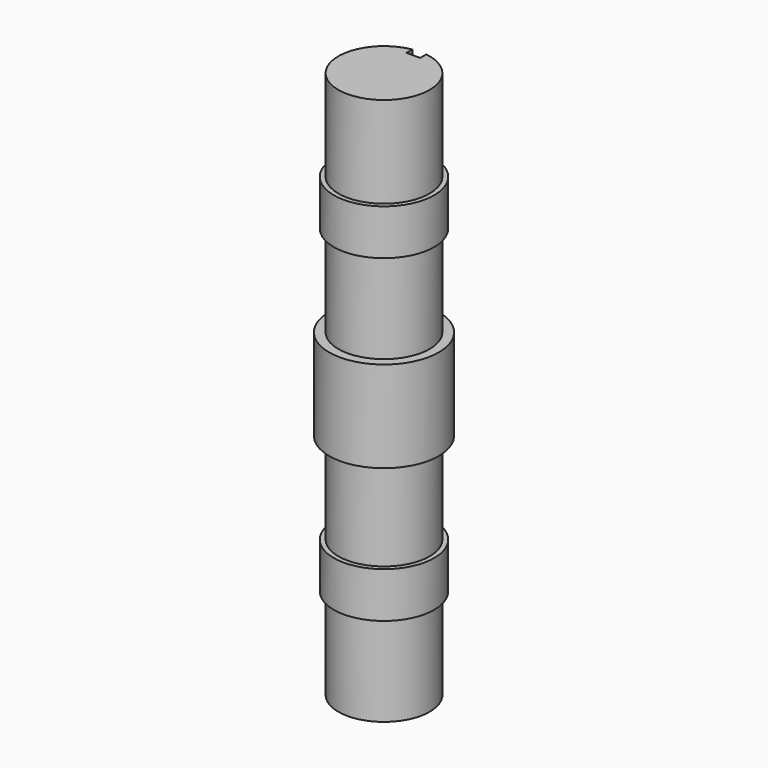
from build123d import *

# Parameters (mm, degrees)
F3_DEPTH = 50
F4_R     = 5


# Not quite as in the source:
# - a pattern or mirror of a feature is missing from the dataset's text; its kind, count and spacing are read off the source's solid


with BuildPart() as f1:
    # F0 (on Right) → F1 (revolve)
    with BuildSketch(Plane.YZ):
        Polygon((-55, -150), (-55, -200), (-50, -200), (-50, -300), (0, -300), (0, 300), (-50, 300), (-50, 200), (-55, 200), (-55, 150), (-50, 150), (-50, 50), (-60, 50), (-60, -50), (-50, -50), (-50, -150), align=None)
    revolve(axis=Axis((0, 0, 0), (0, 0, -1)))

    # F2 (on face) → F3 (cut)
    with BuildSketch(Plane(origin=(0, 0, -300), x_dir=(1, 0, 0), z_dir=(0, 0, -1))):
        with BuildLine():
            Line((-8.3391469531, -41.2996818255), (-8.3391469531, -49.2996818255))
            ThreePointArc((-8.3391469531, -49.2996818255), (-0.8487525257, -49.9927956725), (6.6608530469, -49.5543442766))
            Line((6.6608530469, -49.5543442766), (6.6608530469, -41.2996818255))
            Line((6.6608530469, -41.2996818255), (-8.3391469531, -41.2996818255))
        make_face()
    f3 = extrude(amount=-F3_DEPTH, mode=Mode.SUBTRACT)

    # F3_copies: F3 across plane
    add(f3.mirror(Plane.XY), mode=Mode.SUBTRACT)

    # F4
    f4_edges = [f1.edges().sort_by_distance(p)[0] for p in [
        (6.660853, 45.427013, -250),
        (-8.339147, 45.299682, -250),
        (6.660853, 45.427013, 250),
        (-8.339147, 45.299682, 250),
    ]]
    fillet(f4_edges, radius=F4_R)


solid = f1.part
